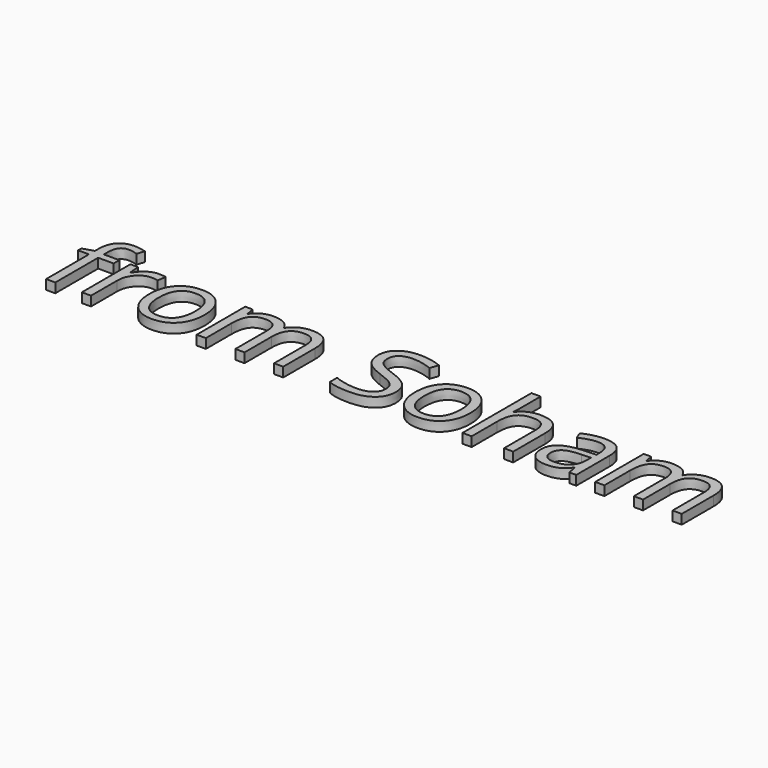
from build123d import *

# Parameters (mm, degrees)
F0_TEXT_SIZE = 301.5562685
F1_DEPTH     = 25.4


# Not quite as in the source:
# - Text() gives the source's letters only with a copy of the font that has no kerning and outlines rounded to 1/6400 em; it was checked with that copy


with BuildPart() as f1:
    # F0 (on Top) → F1 (new body)
    with BuildSketch(Plane.XY):
        with Locations((117.4072548747, -281.3529968262)):
            Text('from Soham', F0_TEXT_SIZE, font='Open Sans', text_align=(TextAlign.LEFT, TextAlign.BOTTOM))
    extrude(amount=F1_DEPTH)


solid = f1.part
